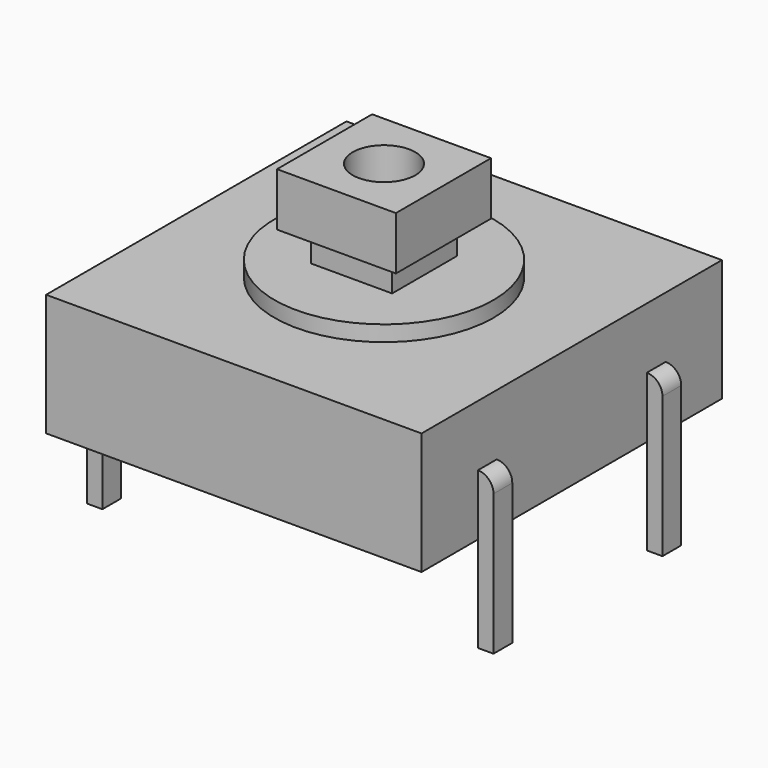
from build123d import *

# Parameters (mm, degrees)
F0_W      = 12
F0_H      = 12
F0_R      = 3.5
F0_W_2    = 3.8
F0_H_2    = 3.8
F0_W_3    = 2.6
F0_H_3    = 2.6
F1_DEPTH  = 3.9
F2_DEPTH  = 0.5
F3_DEPTH  = 1.5
F4_R      = 1
F5_DEPTH  = 3
F6_W      = 3.8
F6_H      = 3.8
F6_W_2    = 2.6
F6_H_2    = 2.6
F7_DEPTH  = 1.7
F8_R      = 1
F9_DEPTH  = 3
F10_W     = 0.75
F10_H     = 3.05
F10_H_2   = 1.95
F12_DEPTH = 0.5
F13_R     = 0.49999
F11_W     = 0.75
F11_H     = 1.95
F11_H_2   = 3.05
F14_DEPTH = 0.5
F15_R     = 0.49999


# Not quite as in the source:
# - a fillet or chamfer is up to 0.001 mm smaller than in the source, because OpenCascade refuses the exact size


with BuildPart() as f1:
    # F0 (on Top) → F1 (new body)
    with BuildSketch(Plane.XY):
        Rectangle(F0_W, F0_H)
        Circle(F0_R, mode=Mode.SUBTRACT)
        Circle(F0_R)
        Rectangle(F0_W_2, F0_H_2, mode=Mode.SUBTRACT)
        Rectangle(F0_W_2, F0_H_2)
        Rectangle(F0_W_3, F0_H_3, mode=Mode.SUBTRACT)
        Rectangle(F0_W_3, F0_H_3)
    extrude(amount=-F1_DEPTH)

    # F0 (on Top) → F2 (join)
    with BuildSketch(Plane.XY):
        Circle(F0_R)
        Rectangle(F0_W_2, F0_H_2, mode=Mode.SUBTRACT)
        Rectangle(F0_W_2, F0_H_2)
        Rectangle(F0_W_3, F0_H_3, mode=Mode.SUBTRACT)
    extrude(amount=F2_DEPTH)

    # F0 (on Top) → F3 (join)
    with BuildSketch(Plane.XY):
        Rectangle(F0_W_3, F0_H_3)
    extrude(amount=F3_DEPTH)

    # F4 (on face) → F5 (cut)
    with BuildSketch(Plane.XY):
        Circle(F4_R)
    extrude(amount=-F5_DEPTH, mode=Mode.SUBTRACT)

    # F6 (on face) → F7 (join)
    with BuildSketch(Plane.XY.offset(1.5)):
        Rectangle(F6_W, F6_H)
        Rectangle(F6_W_2, F6_H_2, mode=Mode.SUBTRACT)
        Rectangle(F6_W_2, F6_H_2)
    extrude(amount=F7_DEPTH)

    # F8 (on face) → F9 (cut)
    with BuildSketch(Plane.XY.offset(3.2)):
        Circle(F8_R)
    extrude(amount=-F9_DEPTH, mode=Mode.SUBTRACT)

    # F10 (on face) → F12 (join)
    with BuildSketch(Plane.YZ.offset(6)):
        with Locations((-3.375, -5.425)):
            Rectangle(F10_W, F10_H)
        with Locations((-3.375, -2.925)):
            Rectangle(F10_W, F10_H_2)
        with Locations((3.375, -5.425)):
            Rectangle(F10_W, F10_H)
        with Locations((3.375, -2.925)):
            Rectangle(F10_W, F10_H_2)
    extrude(amount=F12_DEPTH)

    # F13 (radius 0.5 in the source; OpenCascade refuses exactly that, so slightly less here)
    f13_edges = [f1.edges().sort_by_distance(p)[0] for p in [
        (6.5, -3.375, -1.95),
        (6.5, 3.375, -1.95),
    ]]
    fillet(f13_edges, radius=F13_R)

    # F11 (on face) → F14 (join)
    with BuildSketch(Plane(origin=(-6, 0, 0), x_dir=(0, -1, 0), z_dir=(-1, 0, 0))):
        with Locations((3.375, -2.925)):
            Rectangle(F11_W, F11_H)
        with Locations((-3.375, -2.925)):
            Rectangle(F11_W, F11_H)
        with Locations((-3.375, -5.425)):
            Rectangle(F11_W, F11_H_2)
        with Locations((3.375, -5.425)):
            Rectangle(F11_W, F11_H_2)
    extrude(amount=F14_DEPTH)

    # F15 (radius 0.5 in the source; OpenCascade refuses exactly that, so slightly less here)
    f15_edges = [f1.edges().sort_by_distance(p)[0] for p in [
        (-6.5, 3.375, -1.95),
        (-6.5, -3.375, -1.95),
    ]]
    fillet(f15_edges, radius=F15_R)


solid = f1.part
